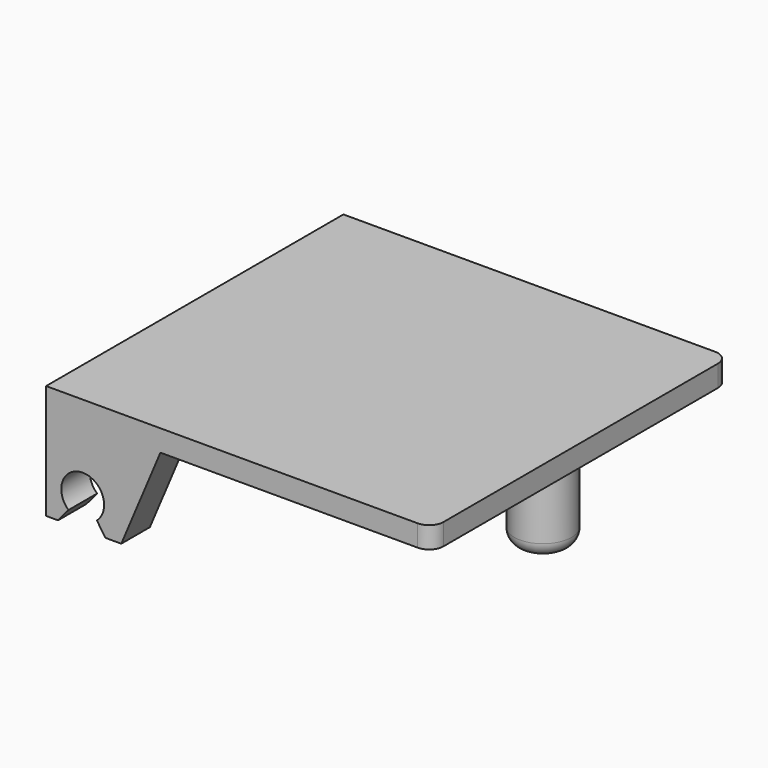
from build123d import *

# Parameters (mm, degrees)
F0_W     = 27
F0_H     = 26
F1_DEPTH = 1.5
F3_DEPTH = 2.5
F5_DEPTH = 26
F7_R     = 2
F8_DEPTH = 10
F9_R     = 1
F10_R    = 1


# Not quite as in the source:
# - a pattern or mirror of a feature is missing from the dataset's text; its kind, count and spacing are read off the source's solid


with BuildPart() as f1:
    # F0 (on Top) → F1 (new body)
    with BuildSketch(Plane.XY):
        with Locations((13.5, 13)):
            Rectangle(F0_W, F0_H)
    extrude(amount=F1_DEPTH)

    # F2 (on Front) → F3 (join)
    with BuildSketch(Plane.XZ):
        with BuildLine():
            Line((2, 0), (0, 0))
            Line((0, 0), (0, -6.5))
            Line((0, -6.5), (0.8364939141, -6.5))
            Line((0.8364939141, -6.5), (1.5690374528, -5.6242691353))
            ThreePointArc((1.5690374528, -5.6242691353), (1.0835712802, -4.2466571982), (2, -3.1092696409))
            Line((2, -3.1092696409), (2, 0))
        make_face()
        with BuildLine():
            Line((8, 0), (3, 0))
            Line((3, 0), (3, -3.0653657134))
            ThreePointArc((3, -3.0653657134), (3.7676272431, -3.6075221422), (4.0620223023, -4.5))
            ThreePointArc((4.0620223023, -4.5), (3.9294061684, -5.1166533571), (3.5550071518, -5.6242691353))
            Line((3.5550071518, -5.6242691353), (4.1543185927, -6.5))
            Line((4.1543185927, -6.5), (5.2601844187, -6.5))
            Line((5.2601844187, -6.5), (8, 0))
        make_face()
        with BuildLine():
            Line((3, 0), (2, 0))
            Line((2, 0), (2, -3.1092696409))
            ThreePointArc((2, -3.1092696409), (2.4962297898, -3.0014435795), (3, -3.0653657134))
            Line((3, -3.0653657134), (3, 0))
        make_face()
    f3 = extrude(amount=-F3_DEPTH)

    # F3_copies: F3 across plane
    add(f3.mirror(Plane.ZX.offset(13)))

    # F4 (on Front) → F5 (join, through all)
    with BuildSketch(Plane.XZ):
        Polygon((2, 0), (0, 0), (0, -4), align=None)
    extrude(amount=-F5_DEPTH)

    # F7 (on face) → F8 (join)
    with BuildSketch(Plane(origin=(0, 0, 0), x_dir=(1, 0, 0), z_dir=(0, 0, -1))):
        with Locations((19, -19.7)):
            Circle(F7_R)
    extrude(amount=F8_DEPTH)

    # F9
    f9_edges = [f1.edges().sort_by_distance(p)[0] for p in [
        (17, 19.7, 0),
        (17, 19.7, -10),
    ]]
    fillet(f9_edges, radius=F9_R)

    # F10
    f10_edges = [f1.edges().sort_by_distance(p)[0] for p in [
        (27, 26, 0.75),
        (27, 0, 0.75),
    ]]
    fillet(f10_edges, radius=F10_R)


solid = f1.part
